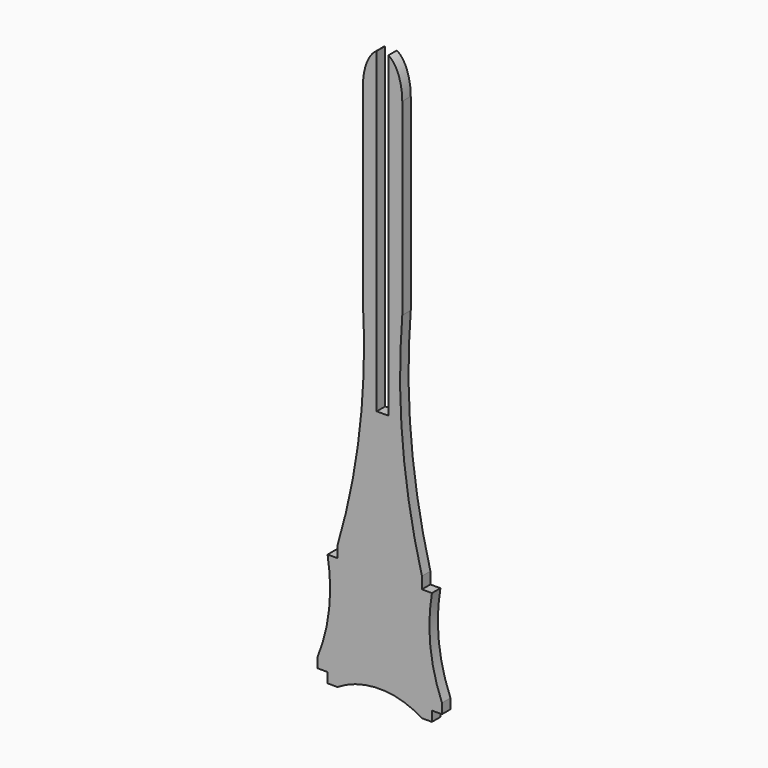
from build123d import *

# Parameters (mm, degrees)
F1_DEPTH = 3.175


# Not quite as in the source:
# - a length typed as a fraction of an inch, garbled in the dataset ("3 / 203.2 mm" for 3/8 in), is restored


with BuildPart() as f1:
    # F0 (on Front) → F1 (new body)
    with BuildSketch(Plane.XZ):
        with BuildLine():
            add(Edge.make_bspline(
                [(-1.75, 126.1528220874), (-5.9, 123.6896499738), (-5.9, 115.3852411336)],
                knots=[3.4427337756, 3.4427337756, 3.4427337756, 4.7123889804, 4.7123889804, 4.7123889804], degree=2, weights=[1, 0.8051739469, 1]))
            Line((-5.9, 115.3852411336), (-1.75, 115.3852411336))
            Line((-1.75, 115.3852411336), (-1.75, 126.1528220874))
        make_face()
        with BuildLine():
            add(Edge.make_bspline(
                [(-5.9, 115.3852411336), (-5.9, 107.0808322935), (-1.75, 104.6176601799)],
                knots=[4.7123889804, 4.7123889804, 4.7123889804, 5.9820441852, 5.9820441852, 5.9820441852], degree=2, weights=[1, 0.8051739469, 1]))
            Line((-5.9, 115.3852411336), (-5.9, 79.8345449512))
            Line((-5.9, 79.8345449512), (-5.9, 58.9576361328))
            ThreePointArc((-5.9, 58.9576361328), (-6.7793812573, 25.2130721087), (-13.4661033603, -7.8740350493))
            Line((-13.4661033603, -7.8740350493), (11.7832735849, -7.8740350493))
            ThreePointArc((11.7832735849, -7.8740350493), (5.9964918029, 25.2913389557), (5.9, 58.9576361328))
            Line((5.9, 58.9576361328), (5.9, 79.8345449512))
            Line((5.9, 79.8345449512), (5.9, 115.3852411336))
            add(Edge.make_bspline(
                [(1.75, 104.6176601799), (5.9, 107.0808322935), (5.9, 115.3852411336)],
                knots=[0.301141122, 0.301141122, 0.301141122, 1.5707963268, 1.5707963268, 1.5707963268], degree=2, weights=[1, 0.8051739469, 1]))
            Line((1.75, 104.6176601799), (1.75, 31.1528220874))
            Line((1.75, 31.1528220874), (-1.75, 31.1528220874))
            Line((-1.75, 31.1528220874), (-1.75, 104.6176601799))
        make_face()
        with BuildLine():
            Line((-1.75, 115.3852411336), (-5.9, 115.3852411336))
            add(Edge.make_bspline(
                [(-5.9, 115.3852411336), (-5.9, 107.0808322935), (-1.75, 104.6176601799)],
                knots=[4.7123889804, 4.7123889804, 4.7123889804, 5.9820441852, 5.9820441852, 5.9820441852], degree=2, weights=[1, 0.8051739469, 1]))
            Line((-1.75, 104.6176601799), (-1.75, 115.3852411336))
        make_face()
        with BuildLine():
            Line((1.75, 126.1528220874), (1.75, 115.3852411336))
            Line((1.75, 115.3852411336), (5.9, 115.3852411336))
            add(Edge.make_bspline(
                [(5.9, 115.3852411336), (5.9, 123.6896499738), (1.75, 126.1528220874)],
                knots=[1.5707963268, 1.5707963268, 1.5707963268, 2.8404515316, 2.8404515316, 2.8404515316], degree=2, weights=[1, 0.8051739469, 1]))
        make_face()
        with BuildLine():
            Line((5.9, 115.3852411336), (1.75, 115.3852411336))
            Line((1.75, 115.3852411336), (1.75, 104.6176601799))
            add(Edge.make_bspline(
                [(1.75, 104.6176601799), (5.9, 107.0808322935), (5.9, 115.3852411336)],
                knots=[0.301141122, 0.301141122, 0.301141122, 1.5707963268, 1.5707963268, 1.5707963268], degree=2, weights=[1, 0.8051739469, 1]))
        make_face()
        with BuildLine():
            Line((11.7832735849, -7.8740350493), (-13.4661033603, -7.8740350493))
            Line((-13.4661033603, -7.8740350493), (-13.4661033603, -11.3740350493))
            Line((-13.4661033603, -11.3740350493), (-16.4661033603, -11.3740350493))
            ThreePointArc((-16.4661033603, -11.3740350493), (-15.9973063906, -25.5681128526), (-19.4661033603, -39.3397889622))
            Line((-19.4661033603, -39.3397889622), (-19.4661033603, -42.3397889622))
            Line((-19.4661033603, -42.3397889622), (-16.5214760231, -42.3397889622))
            Line((-16.5214760231, -42.3397889622), (-16.5214760231, -45.3397889622))
            Line((-16.5214760231, -45.3397889622), (-13.5214760231, -45.3397889622))
            ThreePointArc((-13.5214760231, -45.3397889622), (-0.8691012191, -41.7016149524), (11.7832735849, -45.3397889622))
            Line((11.7832735849, -45.3397889622), (14.7832735849, -45.3397889622))
            Line((14.7832735849, -45.3397889622), (14.7832735849, -42.3397889622))
            Line((14.7832735849, -42.3397889622), (17.7832735849, -42.3397889622))
            Line((17.7832735849, -42.3397889622), (17.7832735849, -39.3397889622))
            ThreePointArc((17.7832735849, -39.3397889622), (14.302318759, -25.5694170752), (14.7832735849, -11.3740350493))
            Line((14.7832735849, -11.3740350493), (11.7832735849, -11.3740350493))
            Line((11.7832735849, -11.3740350493), (11.7832735849, -7.8740350493))
        make_face()
    extrude(amount=F1_DEPTH)


solid = f1.part
